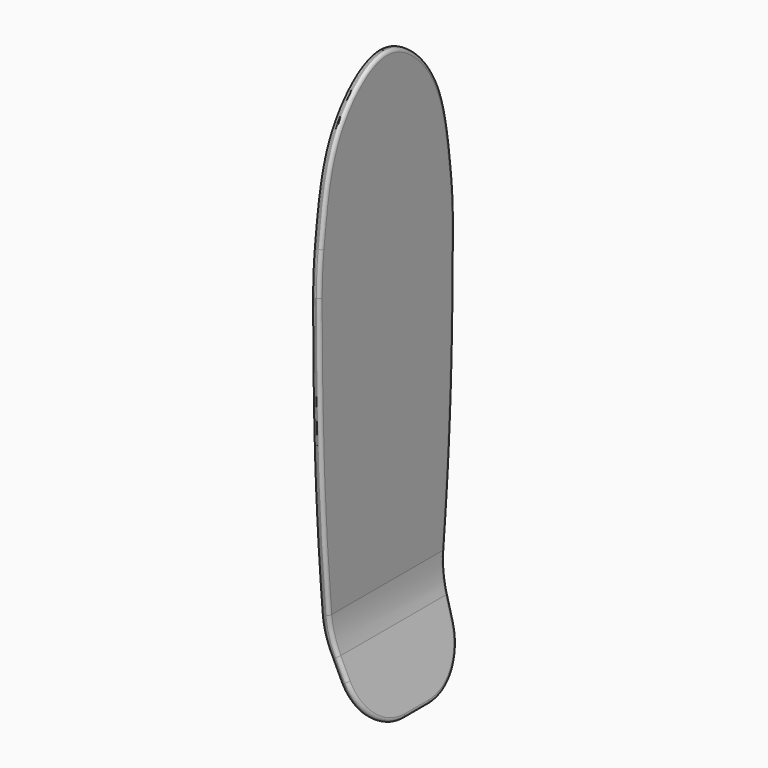
from build123d import *

# Parameters (mm, degrees)
F0_W        = 7.9375
F0_H        = 474.98
F1_DEPTH    = 82.55
F2_W        = 249.0210533142
F2_H        = 601.2149453163
F3_DEPTH    = 50.8
F4_R        = 101.6
F5_T1_DEPTH = 113.7057971067
F6_R        = 101.6
F7_T1_DEPTH = 236.6748680094
F8_R        = 3.175
F9_R        = 3.175


# Not quite as in the source:
# - a fillet or chamfer that OpenCascade refuses, or shapes differently, is made with other operations: its cross-section is extruded or revolved along the edge and cut away or added


with BuildPart() as f1:
    # F0 (on Front) → F1 (new body, symmetric)
    with BuildSketch(Plane.XZ):
        with Locations((0, 41.91)):
            Rectangle(F0_W, F0_H)
        Polygon((36.0391393447, -283.6926705576), (3.96875, -195.58), (-3.96875, -195.58), (29.030150461, -286.2437338836), align=None)
    extrude(amount=F1_DEPTH, both=True)

    # F2 (on Right) → F3 (cut, symmetric)
    with BuildSketch(Plane.YZ):
        with Locations((-6.6651701927, 4.6745538712)):
            Rectangle(F2_W, F2_H)
        with BuildLine():
            add(Edge.make_bspline(
                [(0, 279.4), (-20.7233820111, 279.4), (-68.9412884426, 237.5002619977), (-76.1581808329, 182.61256814), (-82.55, 119.7428571429)],
                knots=[0, 0, 0, 0, 0.4198453869, 1, 1, 1, 1], degree=3))
            add(Edge.make_bspline(
                [(0, 279.4), (20.7233820111, 279.4), (68.9412884426, 237.5002619977), (76.1581808329, 182.61256814), (82.55, 119.7428571429)],
                knots=[0, 0, 0, 0, 0.4198453869, 1, 1, 1, 1], degree=3))
            add(Edge.make_bspline(
                [(82.55, 119.7428571429), (82.55, -49.9441474676), (77.7139365673, -122.4599406123), (60.325, -279.4)],
                knots=[0, 0, 0, 0, 399.7611424753, 399.7611424753, 399.7611424753, 399.7611424753], degree=3))
            Line((60.325, -279.4), (-60.325, -279.4))
            add(Edge.make_bspline(
                [(-82.55, 119.7428571429), (-82.55, -49.9441474676), (-77.7139365673, -122.4599406123), (-60.325, -279.4)],
                knots=[0, 0, 0, 0, 399.7611424753, 399.7611424753, 399.7611424753, 399.7611424753], degree=3))
        make_face(mode=Mode.SUBTRACT)
    extrude(amount=F3_DEPTH, both=True, mode=Mode.SUBTRACT)

    # F4
    f4_edges = [f1.edges().sort_by_distance(p)[0] for p in [
        (-3.96875, 0, -195.58),
    ]]
    fillet(f4_edges, radius=F4_R)

    # F5: fillet of radius 381 on 2 edges, made by hand

    # F5_s2 → F5_t1 (cut)
    with BuildSketch(Plane.YZ.offset(-54.8685235533)):
        with BuildLine():
            ThreePointArc((-82.5249358409, 99.134870303), (-81.9863128344, 120.3844062232), (-80.2634645878, 141.5708331397))
            Line((-80.2634645878, 141.5708331397), (-118.1374329239, 145.7170133739))
            ThreePointArc((-118.1374329239, 145.7170133739), (-119.3216382771, 134.6141833434), (-120.454845274, 123.5965557317))
            Line((-120.454845274, 123.5965557317), (-120.65024, 119.7428571429))
            ThreePointArc((-120.65024, 119.7428571429), (-120.6440614916, 109.3925923013), (-120.6250513022, 99.0374542536))
            Line((-120.6250513022, 99.0374542536), (-82.5249358409, 99.134870303))
        make_face()
        with BuildLine():
            ThreePointArc((82.5249358409, 99.134870303), (81.9863128344, 120.3844062232), (80.2634645878, 141.5708331397))
            Line((80.2634645878, 141.5708331397), (118.1374329239, 145.7170133739))
            ThreePointArc((118.1374329239, 145.7170133739), (119.3216382771, 134.6141833435), (120.454845274, 123.5965557317))
            Line((120.454845274, 123.5965557317), (120.65024, 119.7428571429))
            ThreePointArc((120.65024, 119.7428571429), (120.6440614916, 109.3925923013), (120.6250513022, 99.0374542536))
            Line((120.6250513022, 99.0374542536), (82.5249358409, 99.134870303))
        make_face()
    extrude(amount=F5_T1_DEPTH, mode=Mode.SUBTRACT)

    # F6
    f6_edges = [f1.edges().sort_by_distance(p)[0] for p in [
        (3.96875, 0, -195.58),
    ]]
    fillet(f6_edges, radius=F6_R)

    # F7: fillet of radius 50.8 on 2 edges, made by hand

    # F7_s2 → F7_t1 (cut)
    with BuildSketch(Plane.YZ.offset(-87.8294489685)):
        with BuildLine():
            ThreePointArc((65.252280187, -233.9186494163), (48.7193130034, -266.3549863509), (14.7300185071, -279.4004))
            Line((14.7300185071, -279.4004), (14.7300185071, -284.4805568784))
            ThreePointArc((14.7300185071, -284.4805568784), (37.5275092536, -284.4801568784), (60.325, -284.4801568784))
            Line((60.325, -284.4801568784), (65.3742575438, -279.9594570276))
            ThreePointArc((65.3742575438, -279.9594570276), (67.8697420419, -257.2104585154), (70.304506355, -234.4506312364))
            Line((70.304506355, -234.4506312364), (65.252280187, -233.9186494163))
        make_face()
        with BuildLine():
            ThreePointArc((-14.7300185071, -279.4004), (-48.7193130034, -266.3549863509), (-65.252280187, -233.9186494163))
            Line((-65.252280187, -233.9186494163), (-70.304506355, -234.4506312364))
            ThreePointArc((-70.304506355, -234.4506312364), (-67.8697420419, -257.2104585154), (-65.3742575438, -279.9594570276))
            Line((-65.3742575438, -279.9594570276), (-60.325, -284.4801568784))
            ThreePointArc((-60.325, -284.4801568784), (-37.5275092536, -284.4801568784), (-14.7300185071, -284.4805568784))
            Line((-14.7300185071, -284.4805568784), (-14.7300185071, -279.4004))
        make_face()
    extrude(amount=F7_T1_DEPTH, mode=Mode.SUBTRACT)

    # F8
    f8_edges = [f1.edges().sort_by_distance(p)[0] for p in [
        (3.96875, -80.126107, -39.131404),
        (3.96875, 0, -177.665179),
        (3.96875, -81.987895, 120.3547),
        (3.96875, 80.126107, -39.131404),
        (3.96875, -62.837845, 225.644715),
        (3.96875, 81.987895, 120.3547),
        (3.96875, 62.837845, 225.644715),
        (29.557145, 49.235816, -265.883537),
        (34.476735, 0, -279.4),
        (29.557145, -49.235816, -265.883537),
        (14.046406, -66.363849, -223.268133),
        (10.09598, 0, -212.414425),
        (14.046406, 66.363849, -223.268133),
    ]]
    fillet(f8_edges, radius=F8_R)

    # F9
    f9_edges = [f1.edges().sort_by_distance(p)[0] for p in [
        (-3.96875, 0, -177.665179),
        (-3.96875, 80.126107, -39.131404),
        (-3.96875, 81.987895, 120.3547),
        (-3.96875, 62.837845, 225.644715),
        (-3.96875, -62.837845, 225.644715),
        (-3.96875, -81.987895, 120.3547),
        (-3.96875, -80.126107, -39.131404),
        (21.619645, -49.235816, -265.883538),
        (26.539235, 0, -279.4),
        (21.619645, 49.235816, -265.883538),
        (6.108907, 66.363849, -223.268134),
        (2.15848, 0, -212.414425),
        (6.108907, -66.363849, -223.268134),
        (1.02233, 67.808842, -209.117946),
        (-2.971517, 69.512345, -191.865292),
        (1.02233, -67.808842, -209.117946),
        (-2.971517, -69.512345, -191.865292),
    ]]
    fillet(f9_edges, radius=F9_R)


solid = f1.part
